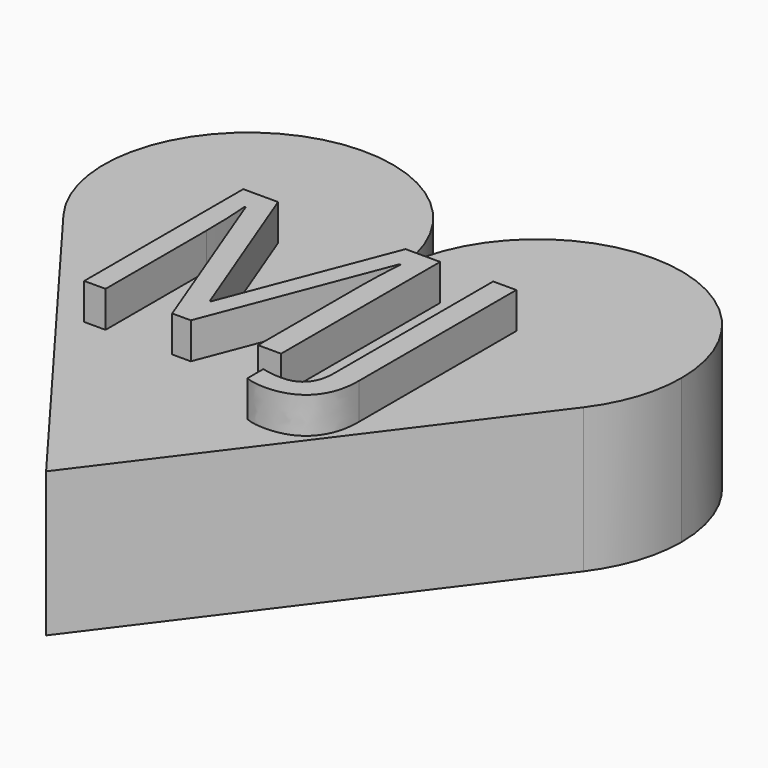
from build123d import *

# Parameters (mm, degrees)
F1_DEPTH     = 25.4
F2_TEXT_SIZE = 48.9719315535
F3_DEPTH     = 6.35


# Not quite as in the source:
# - Text() gives the source's letters only with a copy of the font that has no kerning and outlines rounded to 1/6400 em; it was checked with that copy


with BuildPart() as f1:
    # F0 (on Top) → F1 (new body)
    with BuildSketch(Plane.XY):
        with BuildLine():
            Line((-25.4, 76.2), (0, 76.2))
            ThreePointArc((0, 76.2), (-33.4321852568, 100.2965557705), (-45.72, 60.96))
            ThreePointArc((-45.72, 60.96), (-36.7592253257, 53.4815493486), (-25.4, 50.8))
            Line((-25.4, 50.8), (-25.4, 76.2))
        make_face()
        with BuildLine():
            ThreePointArc((50.8, 76.2), (25.4, 101.6), (0, 76.2))
            ThreePointArc((0, 76.2), (17.3678147432, 52.1034442295), (45.72, 60.96))
            ThreePointArc((45.72, 60.96), (49.4965557705, 68.1678147432), (50.8, 76.2))
        make_face()
        with BuildLine():
            Line((0, 76.2), (0, 0))
            Line((0, 0), (45.72, 60.96))
            ThreePointArc((45.72, 60.96), (17.3678147432, 52.1034442295), (0, 76.2))
        make_face()
        with BuildLine():
            Line((-45.72, 60.96), (-25.4, 33.8666666667))
            Line((-25.4, 33.8666666667), (-25.4, 50.8))
            ThreePointArc((-25.4, 50.8), (-36.7592253257, 53.4815493486), (-45.72, 60.96))
        make_face()
        with BuildLine():
            Line((-25.4, 33.8666666667), (0, 0))
            Line((0, 0), (0, 76.2))
            ThreePointArc((0, 76.2), (-7.4394877579, 58.2394877579), (-25.4, 50.8))
            Line((-25.4, 50.8), (-25.4, 33.8666666667))
        make_face()
        with BuildLine():
            ThreePointArc((-25.4, 50.8), (-7.4394877579, 58.2394877579), (0, 76.2))
            Line((0, 76.2), (-25.4, 76.2))
            Line((-25.4, 76.2), (-25.4, 50.8))
        make_face()
    extrude(amount=F1_DEPTH)

    # F2 (on face) → F3 (join)
    with BuildSketch(Plane.XY.offset(25.4)):
        with Locations((-28.4690093249, 37.9586790999)):
            Text('MJ', F2_TEXT_SIZE, font='Open Sans', text_align=(TextAlign.LEFT, TextAlign.BOTTOM))
    extrude(amount=F3_DEPTH)


solid = f1.part
